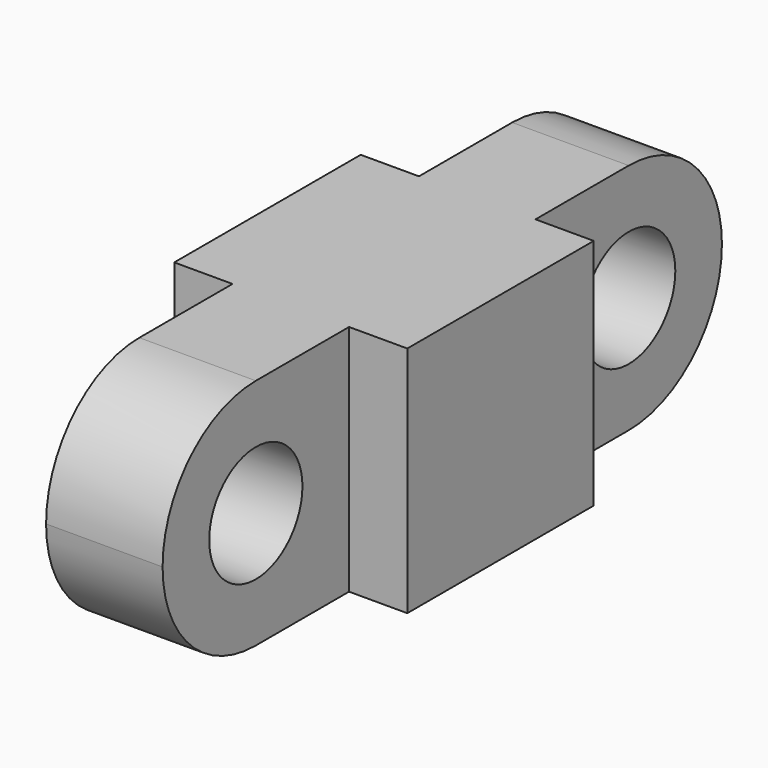
from build123d import *

# Parameters (mm, degrees)
F1_DEPTH = 40
F2_R     = 10
F3_DEPTH = 20
F4_R     = 10
F5_DEPTH = 20
F6_R     = 19.99999
F7_R     = 19.99999


# Not quite as in the source:
# - a fillet or chamfer is up to 0.001 mm smaller than in the source, because OpenCascade refuses the exact size


with BuildPart() as f1:
    # F0 (on Top) → F1 (new body)
    with BuildSketch(Plane.XY):
        Polygon((0, 0), (0, 120), (-10, 120), (-10, 80), (-20, 80), (-20, 40), (-10, 40), (-10, 0), align=None)
        Polygon((10, 120), (0, 120), (0, 0), (10, 0), (10, 40), (20, 40), (20, 80), (10, 80), align=None)
    extrude(amount=F1_DEPTH)

    # F2 (on face) → F3 (cut, through all)
    with BuildSketch(Plane.YZ.offset(10)):
        with Locations((20, 20)):
            Circle(F2_R)
    extrude(amount=-F3_DEPTH, mode=Mode.SUBTRACT)

    # F4 (on face) → F5 (cut, through all)
    with BuildSketch(Plane.YZ.offset(10)):
        with Locations((100, 20)):
            Circle(F4_R)
    extrude(amount=-F5_DEPTH, mode=Mode.SUBTRACT)

    # F6 (radius 20 in the source; OpenCascade refuses exactly that, so slightly less here)
    f6_edges = [f1.edges().sort_by_distance(p)[0] for p in [
        (0, 120, 0),
        (0, 120, 40),
    ]]
    fillet(f6_edges, radius=F6_R)

    # F7 (radius 20 in the source; OpenCascade refuses exactly that, so slightly less here)
    f7_edges = [f1.edges().sort_by_distance(p)[0] for p in [
        (0, 0, 40),
        (0, 0, 0),
    ]]
    fillet(f7_edges, radius=F7_R)


solid = f1.part
